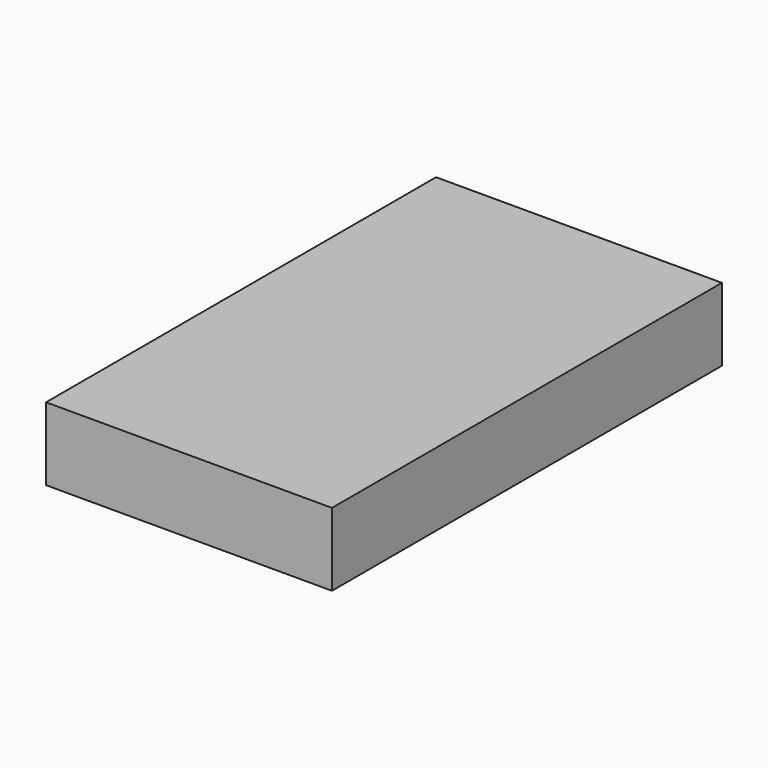
from build123d import *

# Parameters (mm, degrees)
F0_W         = 99.4600877166
F0_H         = 169.5871688426
F1_DEPTH     = 25.4
F2_TEXT_SIZE = 7.239690033
F3_DEPTH     = 12.7


# Not quite as in the source:
# - Text() gives the source's letters only with a copy of the font that has no kerning and outlines rounded to 1/6400 em; it was checked with that copy


with BuildPart() as f1:
    # F0 (on Top) → F1 (new body)
    with BuildSketch(Plane.XY):
        with Locations((0, -4.0252190083)):
            Rectangle(F0_W, F0_H)
    extrude(amount=F1_DEPTH)

    # F2 (on face) → F3 (join)
    with BuildSketch(Plane(origin=(0, 0, 0), x_dir=(1, 0, 0), z_dir=(0, 0, -1))):
        with Locations((-45.6774377198, 48.7931988571)):
            Text('Wesley Koh Gwee Sing', F2_TEXT_SIZE, font='Open Sans', text_align=(TextAlign.LEFT, TextAlign.BOTTOM))
    extrude(amount=F3_DEPTH)


solid = f1.part
